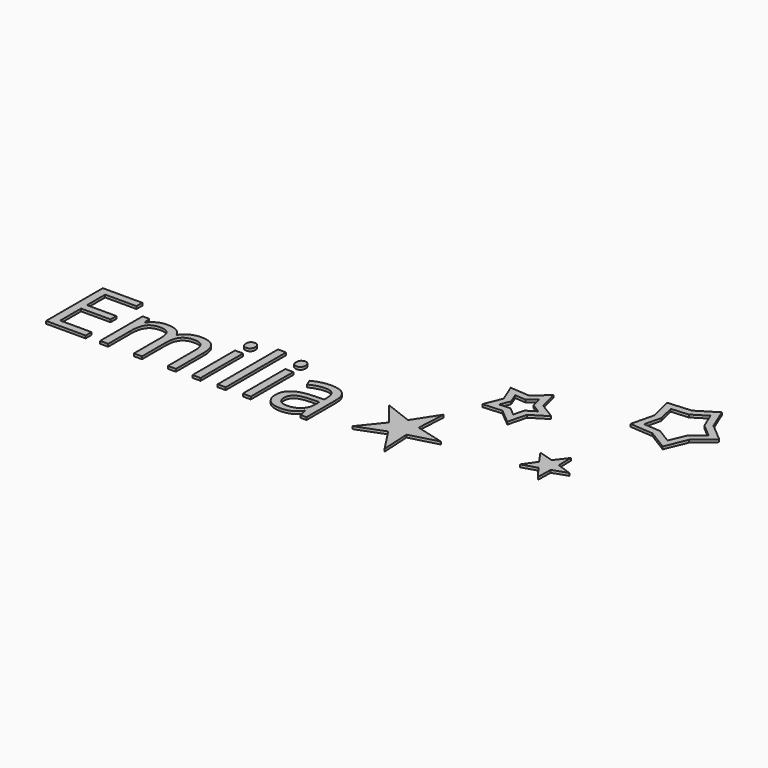
from build123d import *

# Parameters (mm, degrees)
F0_TEXT_SIZE = 11.4894810659
F1_DEPTH     = 0.3


# Not quite as in the source:
# - Text() gives the source's letters only with a copy of the font that has no kerning and outlines rounded to 1/6400 em; it was checked with that copy


with BuildPart() as f1:
    # F0 (on Top) → F1 (new body)
    with BuildSketch(Plane.XY):
        Polygon((45.5197678753, 19.2148680571), (42.8062423837, 19.0067321436), (43.4468188584, 16.3616985083), (42.8062423837, 13.7166648729), (45.5197678753, 13.5085289594), (47.8373953331, 12.0819441849), (48.8738698415, 14.5983427514), (50.9468188584, 16.3616985083), (48.8738698415, 18.1250542651), (47.8373953331, 20.6414528316), align=None)
        Polygon((47.4558552841, 19.467193304), (48.2079466306, 17.641232732), (49.7121293236, 16.3616985083), (48.2079466306, 15.0821642845), (47.4558552841, 13.2562037126), (45.7741279079, 14.2913686445), (43.8051272001, 14.4423971726), (44.2699452149, 16.3616985083), (43.8051272001, 18.2809998439), (45.7741279079, 18.4320283721), align=None, mode=Mode.SUBTRACT)
        Polygon((32.15595247, 12.3196945685), (29.9424269785, 12.4748299189), (30.7739864588, 10.4175815359), (29.9424269785, 8.3603331529), (32.15595247, 8.5154685033), (33.8555459391, 7.0888837288), (34.3920204475, 9.2420110313), (36.2739864588, 10.4175815359), (34.3920204475, 11.5931520405), (33.8555459391, 13.7462793429), align=None)
        Polygon((33.3889164299, 12.3101413844), (33.6939336388, 11.0859622857), (34.7639416466, 10.4175815359), (33.6939336388, 9.7492007861), (33.3889164299, 8.5250216874), (32.4225979039, 9.3361187653), (31.1640788938, 9.2479152238), (31.6368692086, 10.4175815359), (31.1640788938, 11.587247848), (32.4225979039, 11.4990443064), align=None, mode=Mode.SUBTRACT)
        Polygon((41.6785921238, 3.7183704865), (39.9650666323, 4.236777101), (40.9876091182, 2.7673139703), (39.9650666323, 1.2978508395), (41.6785921238, 1.816257454), (42.7601516042, 0.3896726795), (42.7966261126, 2.179528718), (44.4876091182, 2.7673139703), (42.7966261126, 3.3550992225), (42.7601516042, 5.144955261), align=None)
        Polygon((26.6473156337, 1.7384390408), (23.4702646506, 2.9568879016), (25.6108411252, 0.3118542663), (23.4702646506, -2.333179369), (26.6473156337, -1.1147305081), (28.5014175999, -3.967900057), (28.3243666168, -0.5698236121), (31.6108411252, 0.3118542663), (28.3243666168, 1.1935321448), (28.5014175999, 4.5916085897), align=None)
        with Locations((-12.1212715749, -3.5333816676)):
            Text('Emilia', F0_TEXT_SIZE, font='Open Sans', text_align=(TextAlign.LEFT, TextAlign.BOTTOM))
    extrude(amount=F1_DEPTH)


solid = f1.part
